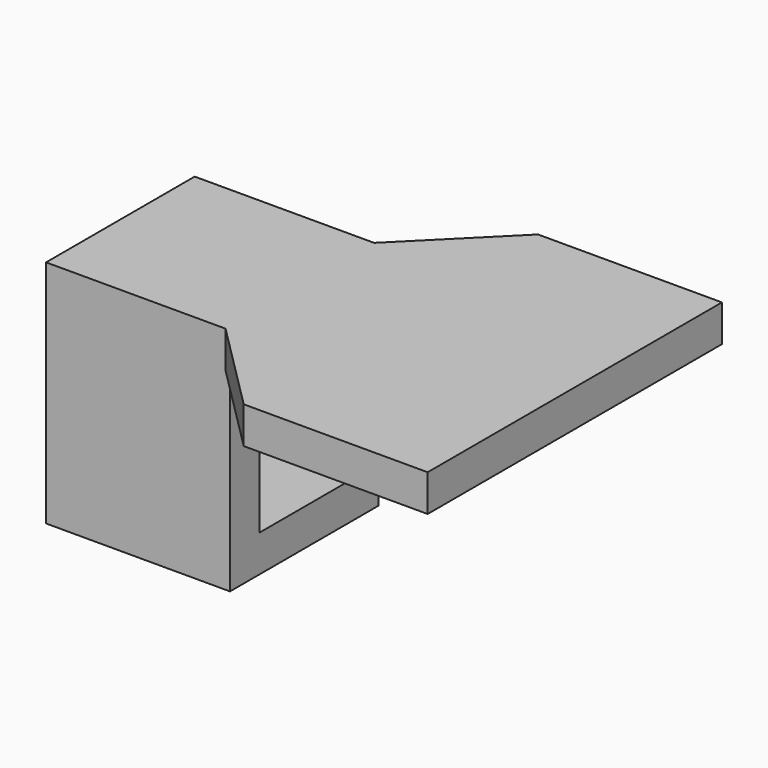
from build123d import *

# Parameters (mm, degrees)
F0_W        = 10.1
F0_H        = 12.5
F0_W_2      = 6.1
F0_H_2      = 8.5
F1_DEPTH    = 10
F2_W        = 15
F2_H        = 2
F3_DEPTH    = 10
F4_T4_DEPTH = 27.7168298797
F4_T9_DEPTH = 27.7168298797


# Not quite as in the source:
# - a fillet or chamfer that OpenCascade refuses, or shapes differently, is made with other operations: its cross-section is extruded or revolved along the edge and cut away or added


with BuildPart() as f1:
    # F0 (on Right) → F1 (new body)
    with BuildSketch(Plane.YZ):
        Rectangle(F0_W, F0_H)
        Rectangle(F0_W_2, F0_H_2, mode=Mode.SUBTRACT)
    extrude(amount=F1_DEPTH)

    # F2 (on Front) → F3 (join, symmetric)
    with BuildSketch(Plane.XZ):
        with Locations((17.2066340968, 5.25)):
            Rectangle(F2_W, F2_H)
    extrude(amount=F3_DEPTH, both=True)

    # F4: chamfer of 5 on 2 edges, made by hand


with BuildPart() as f4_tool2:
    # F4_s3 → F4_t4 (new body)
    with BuildSketch(Plane.XY.offset(19.1084149398)):
        Polygon((14.7066340968, 10), (9.7066340968, 5), (9.7066340968, 10), align=None)
    extrude(amount=-F4_T4_DEPTH)

    split(bisect_by=Plane.XZ.offset(-5.05), keep=Keep.BOTTOM)


with BuildPart() as f1_1:
    add(f1.part)

    # F4_t1: cut F4_tool2
    add(f4_tool2.part, mode=Mode.SUBTRACT)


with BuildPart() as f4_tool7:
    # F4_s8 → F4_t9 (new body)
    with BuildSketch(Plane.XY.offset(19.1084149398)):
        Polygon((9.7066340968, -5), (14.7066340968, -10), (9.7066340968, -10), align=None)
    extrude(amount=-F4_T9_DEPTH)

    split(bisect_by=Plane.XZ.offset(5.05), keep=Keep.TOP)


with BuildPart() as f1_2:
    add(f1_1.part)

    # F4_t6: cut F4_tool7
    add(f4_tool7.part, mode=Mode.SUBTRACT)


solid = f1_2.part
